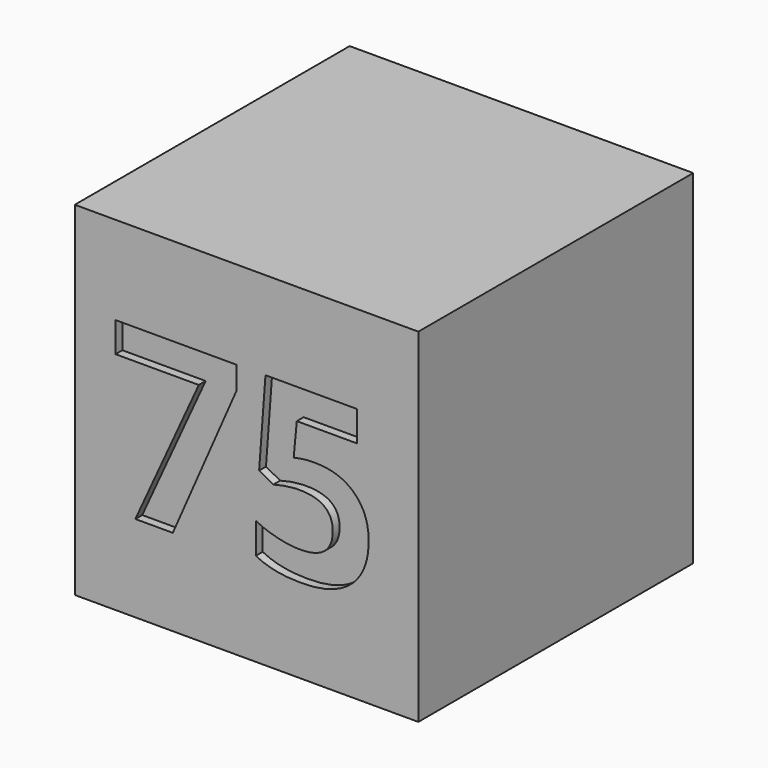
from build123d import *

# Parameters (mm, degrees)
F0_W         = 20
F0_H         = 20
F1_DEPTH     = 10
F2_TEXT_SIZE = 13.7745493678
F3_DEPTH     = 0.5


# Not quite as in the source:
# - Text() gives the source's letters only with a copy of the font that has no kerning and outlines rounded to 1/6400 em; it was checked with that copy


with BuildPart() as f1:
    # F0 (on Top) → F1 (new body, symmetric)
    with BuildSketch(Plane.XY):
        Rectangle(F0_W, F0_H)
    extrude(amount=F1_DEPTH, both=True)

    # F2 (on face) → F3 (cut)
    with BuildSketch(Plane.XZ.offset(10)):
        with Locations((-8, -4.9588377724)):
            Text('75', F2_TEXT_SIZE, font='Open Sans', font_style=FontStyle.BOLD, text_align=(TextAlign.LEFT, TextAlign.BOTTOM))
    extrude(amount=-F3_DEPTH, mode=Mode.SUBTRACT)


solid = f1.part
